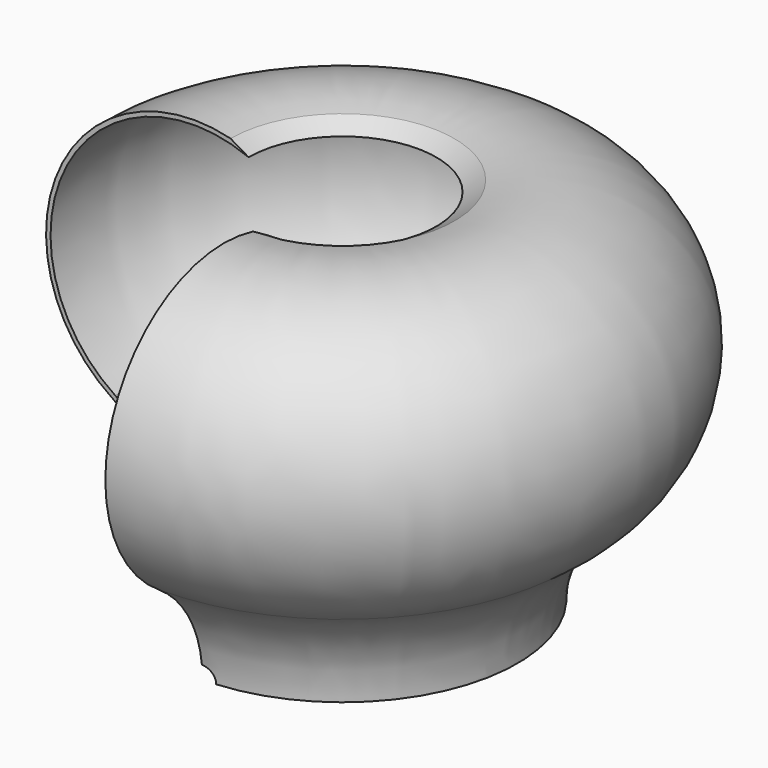
from build123d import *

# Parameters (mm, degrees)
F1_ANGLE = 270
F3_DEPTH = 100.001


# Not quite as in the source:
# - a feature names something its author has since deleted; it is built from what else it names


with BuildPart() as f1:
    # F0 (on Right) → F1 (revolve)
    with BuildSketch(Plane.YZ):
        with BuildLine():
            ThreePointArc((-76.6564003216, 35.4822715112), (-92.9111910846, 98.6026476259), (-31.6640544802, 120.9003686165))
            Line((-31.6640544802, 120.9003686165), (-37.7450487886, 124.4749024837))
            ThreePointArc((-37.7450487886, 124.4749024837), (-95.7605829794, 96.1486735392), (-77.4808250738, 34.2291458878))
            ThreePointArc((-77.4808250738, 34.2291458878), (-63.9346767138, 19.4432539414), (-59.0274766756, 0))
            Line((-59.0274766756, 0), (-57.5274766756, 0))
            ThreePointArc((-57.5274766756, 0), (-62.6143288187, 20.1550695325), (-76.6564003216, 35.4822715112))
        make_face()
    revolve(axis=Axis((0, 0, 76), (0, 0, 1)), revolution_arc=F1_ANGLE)

    # F2 (on Front) → F3 (cut, through all)
    with BuildSketch(Plane.XZ):
        with BuildLine():
            Line((-4.5, 0), (4.5, 0))
            ThreePointArc((4.5, 0), (0, 4.5), (-4.5, 0))
        make_face()
    extrude(amount=F3_DEPTH, mode=Mode.SUBTRACT)


solid = f1.part
